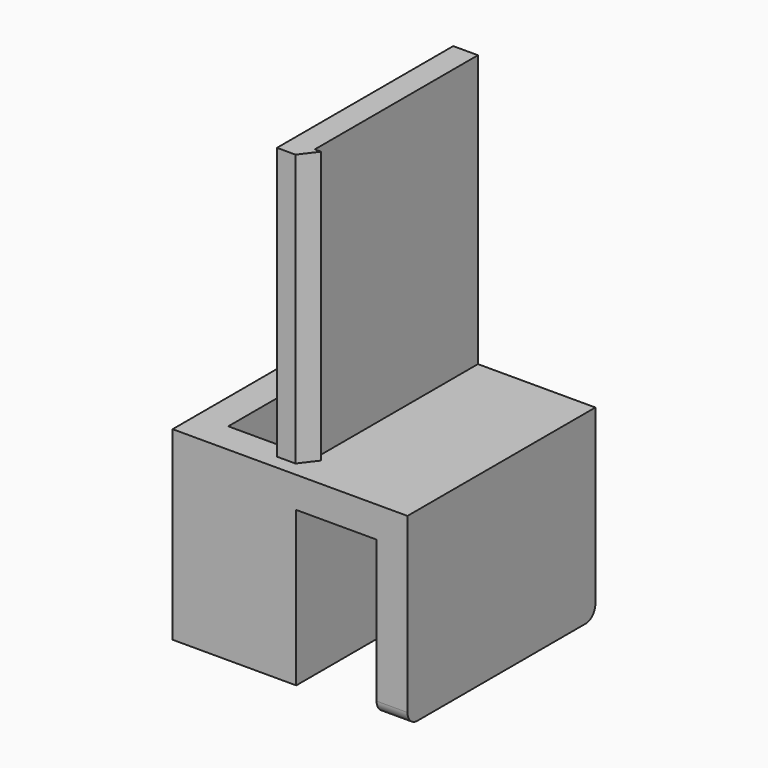
from build123d import *

# Parameters (mm, degrees)
F0_W     = 10
F0_H     = 15
F1_DEPTH = 19
F2_T     = -2.5
F3_DEPTH = 9
F4_T     = -2.5
F5_DEPTH = 25
F6_DEPTH = 25
F8_DEPTH = 22
F9_R     = 1


# Not quite as in the source:
# - two fillets or chamfers of one size are made in one step


with BuildPart() as f1:
    # F0 (on Front) → F1 (new body)
    with BuildSketch(Plane.XZ):
        with Locations((-35.433777729, 22.9624143615)):
            Rectangle(F0_W, F0_H)
    extrude(amount=F1_DEPTH)

    # F2
    f2_openings = [f1.faces().sort_by_distance(p)[0] for p in [
        (-35.433778, 0, 22.962414),
        (-35.433778, -9.5, 30.462414),
    ]]
    offset(amount=F2_T, openings=f2_openings)

    # F3 (add): a face of the model
    f3_faces = [f1.faces().sort_by_distance(p)[0] for p in [
        (-30.433777729, -9.5, 22.9624143615),
    ]]
    extrude(f3_faces, amount=F3_DEPTH)

    # F4: a shell. OpenCascade refuses it in one call, so the cavity is built on its own and cut out:
    # the body offset inwards by the wall thickness, plus a prism from it out through each open face.
    f4_core = offset(f1.part, amount=F4_T, kind=Kind.INTERSECTION, mode=Mode.PRIVATE)
    f4_exits = [f4_core.faces().sort_by_distance(p)[0] for p in [
        (-27.183778, -2.5, 22.962414),
    ]]
    add(f4_core, mode=Mode.SUBTRACT)
    extrude(f4_exits, amount=-F4_T, mode=Mode.SUBTRACT)

    # F5 (cut): a face of the model
    f5_faces = [f1.faces().sort_by_distance(p)[0] for p in [
        (-27.183777729, -16.5, 22.9624143615),
    ]]
    extrude(f5_faces, amount=-F5_DEPTH, mode=Mode.SUBTRACT)

    # F6 (cut): a face of the model
    f6_faces = [f1.faces().sort_by_distance(p)[0] for p in [
        (-27.183777729, -9.5, 17.9624143615),
    ]]
    extrude(f6_faces, amount=-F6_DEPTH, mode=Mode.SUBTRACT)

    # F7 (on face) → F8 (join)
    with BuildSketch(Plane.XY.offset(30.4624143615)):
        Polygon((-30.933777729, 0), (-32.933777729, 0), (-32.933777729, -17.8228756555), (-31.933777729, -17.8228756555), (-31.433777729, -17.8228756555), (-30.433777729, -16.5), (-30.933777729, -16.5), align=None)
    extrude(amount=F8_DEPTH)

    # F9
    f9_edges = [f1.edges().sort_by_distance(p)[0] for p in [
        (-22.683778, 0, 15.462414),
        (-22.683778, -19, 15.462414),
        (-39.183778, 0, 30.462414),
    ]]
    fillet(f9_edges, radius=F9_R)


solid = f1.part
